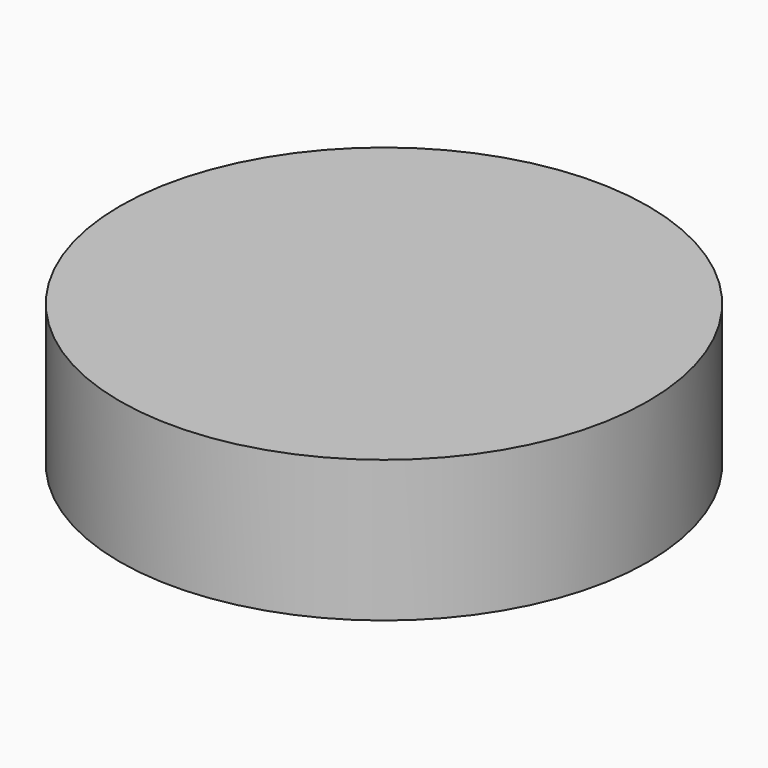
from build123d import *

# Parameters (mm, degrees)
F0_R     = 23.7109
F1_DEPTH = 12.7


# Not quite as in the source:
# - a feature of the source that left no trace in its solid (it failed there, or was rolled back) is left out


with BuildPart() as f1:
    # F0 (on Top) → F1 (new body)
    with BuildSketch(Plane.XY):
        Circle(F0_R)
    extrude(amount=F1_DEPTH)


solid = f1.part
